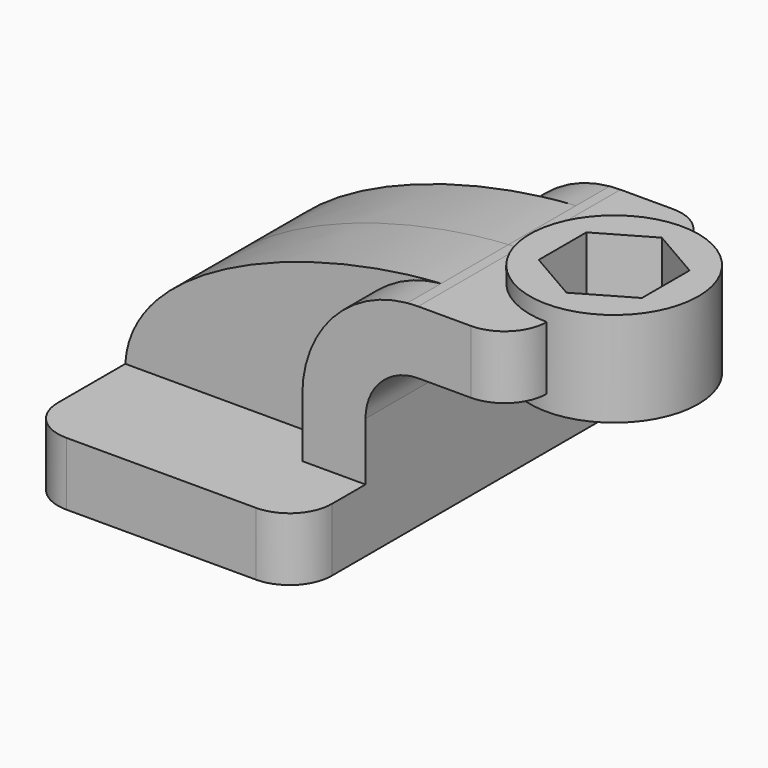
from build123d import *

# Parameters (mm, degrees)
F1_DEPTH = 63.5
F2_DEPTH = 25.4
F0_W     = 25.4
F0_H     = 19.05
F3_DEPTH = 38.1
F6_DEPTH = 91.186
F7_R     = 12.69999


# Not quite as in the source:
# - a fillet or chamfer is up to 0.001 mm smaller than in the source, because OpenCascade refuses the exact size


with BuildPart() as f1:
    # F0 (on Front) → F1 (new body, symmetric)
    with BuildSketch(Plane.XZ):
        Polygon((22.225, 9.525), (-41.275, 9.525), (-41.275, -9.525), (41.275, -9.525), (41.275, 9.525), align=None)
    extrude(amount=F1_DEPTH, both=True)

    # F0 (on Front) → F2 (join, symmetric)
    with BuildSketch(Plane.XZ):
        with BuildLine():
            add(Edge.make_bspline(
                [(-41.275, 9.525), (-39.5856284224, 39.4828766469), (13.870125209, 59.4306981306), (53.8854342407, 61.7722898912)],
                knots=[0, 0, 0, 0, 108.5245810491, 108.5245810491, 108.5245810491, 108.5245810491], degree=3))
            Line((-41.275, 9.525), (22.225, 9.525))
            Line((22.225, 9.525), (22.225, 27.0002))
            ThreePointArc((22.225, 27.0002), (31.3258777096, 50.5133948686), (53.8854342407, 61.7722898912))
        make_face()
    extrude(amount=F2_DEPTH, both=True)

    # F0 (on Front) → F3 (join, symmetric)
    with BuildSketch(Plane.XZ):
        with BuildLine():
            Line((22.225, 27.0002), (22.225, 9.525))
            Line((22.225, 9.525), (41.275, 9.525))
            Line((41.275, 9.525), (41.275, 27.0002))
            ThreePointArc((41.275, 27.0002), (45.9246798487, 38.2255201513), (57.15, 42.8752))
            Line((57.15, 42.8752), (60.325, 42.8752))
            Line((60.325, 42.8752), (60.325, 61.9252))
            Line((60.325, 61.9252), (57.15, 61.9252))
            add(Edge.make_bspline(
                [(53.8854342407, 61.7722898912), (54.9842067368, 61.8365871986), (56.0728453275, 61.8876096574), (57.15, 61.9252)],
                knots=[108.5245810491, 108.5245810491, 108.5245810491, 108.5245810491, 111.5045361635, 111.5045361635, 111.5045361635, 111.5045361635], degree=3))
            ThreePointArc((53.8854342407, 61.7722898912), (31.3258777096, 50.5133948686), (22.225, 27.0002))
        make_face()
        with Locations((73.025, 52.4002)):
            Rectangle(F0_W, F0_H)
    extrude(amount=F3_DEPTH, both=True)

    # F0 (on Front) → F4 (revolve)
    with BuildSketch(Plane.XZ):
        Polygon((85.725, 66.675), (85.725, 61.9252), (85.725, 42.8752), (85.725, 38.1), (111.125, 38.1), (111.125, 66.675), align=None)
    revolve(axis=Axis((85.725, 0, 52.3875), (0, 0, 1)))

    # F5 (on face) → F6 (cut)
    with BuildSketch(Plane.XY.offset(66.675)):
        Polygon((101.2713760138, -8.9757043765), (101.2713760138, 8.9757043765), (85.725, 17.9514087529), (70.1786239862, 8.9757043765), (70.1786239862, -8.9757043765), (85.725, -17.9514087529), align=None)
    extrude(amount=-F6_DEPTH, mode=Mode.SUBTRACT)

    # F7 (radius 12.7 in the source; OpenCascade refuses exactly that, so slightly less here)
    f7_edges = [f1.edges().sort_by_distance(p)[0] for p in [
        (85.725, -38.1, 52.4002),
        (85.725, 38.1, 52.4002),
        (41.275, -63.5, 0),
        (-41.275, -63.5, 0),
        (41.275, 63.5, 0),
    ]]
    fillet(f7_edges, radius=F7_R)


solid = f1.part
